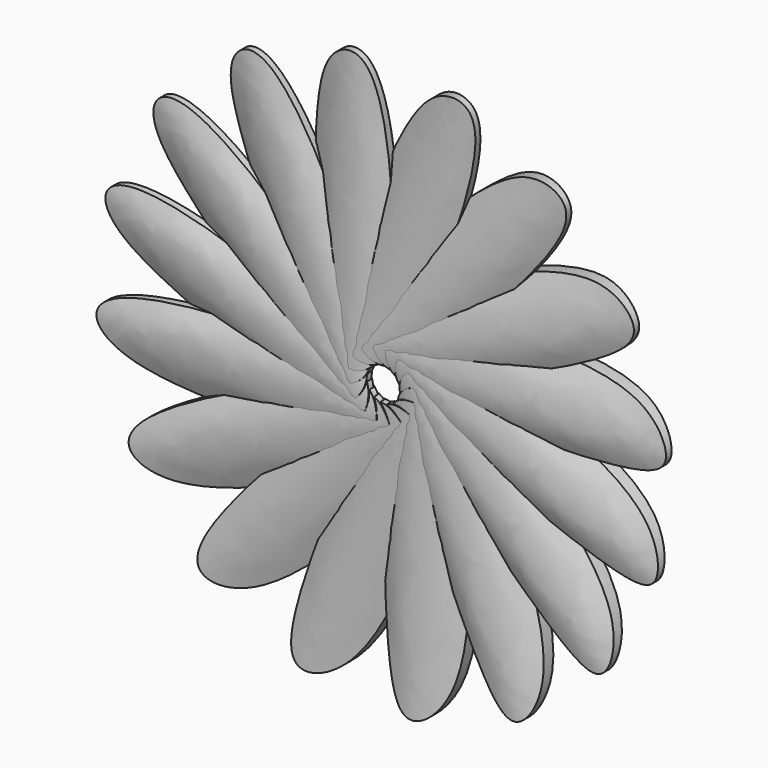
from build123d import *

# Parameters (mm, degrees)
F1_DEPTH = 204
F3_DEPTH = 239
F5_COUNT = 16


with BuildPart() as f1:
    # F0 (on Front) → F1 (new body)
    with BuildSketch(Plane.XZ):
        with BuildLine():
            add(Edge.make_bspline(
                [(-7.4497908354, 168.1414097548), (-10.6516571728, 175.3745122993), (-20.4285228845, 182.9338430563), (-51.5047578624, 156.8177421618), (-47.8448563761, 50.2878389514), (-42.154271715, 4.9962190415), (1.7281079868, -2.3732249511), (4.5337161088, 72.1772189596), (0.5072309671, 150.166282569), (-7.4497908354, 168.1414097548)],
                knots=[0, 0, 0, 0, 0.0807346923, 0.1910522316, 0.4010784068, 0.5334124626, 0.6354068455, 0.7993646083, 1, 1, 1, 1], degree=3))
        make_face()
    extrude(amount=-F1_DEPTH)

    # F2 (on Top) → F3 (intersect)
    with BuildSketch(Plane.XY):
        with BuildLine():
            add(Edge.make_bspline(
                [(39.14796561, 77.6659548283), (39.7631733274, 75.0005164585), (-7.9876774143, -5.9230808558), (-85.7035007244, 65.9992408008), (-85.6405096903, 76.7342301896), (-26.4536337018, 24.2260337862), (10.3763836207, 41.8162409032), (38.6835304134, 79.6781587689), (39.14796561, 77.6659548283)],
                knots=[0, 0, 0, 0, 0.2073158311, 0.4360276951, 0.4754246157, 0.677895944, 0.8434922611, 1, 1, 1, 1], degree=3))
        make_face()
    extrude(amount=F3_DEPTH, mode=Mode.INTERSECT)


with BuildPart() as f5_1:
    # F5: instance of F1
    add(f1.part.rotate(Axis((0, 16.0662084818, 0), (0, 1, 0)), 1 * 360 / F5_COUNT))


with BuildPart() as f5_2:
    # F5: instance of F1
    add(f1.part.rotate(Axis((0, 16.0662084818, 0), (0, 1, 0)), 2 * 360 / F5_COUNT))


with BuildPart() as f5_3:
    # F5: instance of F1
    add(f1.part.rotate(Axis((0, 16.0662084818, 0), (0, 1, 0)), 3 * 360 / F5_COUNT))


with BuildPart() as f5_4:
    # F5: instance of F1
    add(f1.part.rotate(Axis((0, 16.0662084818, 0), (0, 1, 0)), 4 * 360 / F5_COUNT))


with BuildPart() as f5_5:
    # F5: instance of F1
    add(f1.part.rotate(Axis((0, 16.0662084818, 0), (0, 1, 0)), 5 * 360 / F5_COUNT))


with BuildPart() as f5_6:
    # F5: instance of F1
    add(f1.part.rotate(Axis((0, 16.0662084818, 0), (0, 1, 0)), 6 * 360 / F5_COUNT))


with BuildPart() as f5_7:
    # F5: instance of F1
    add(f1.part.rotate(Axis((0, 16.0662084818, 0), (0, 1, 0)), 7 * 360 / F5_COUNT))


with BuildPart() as f5_8:
    # F5: instance of F1
    add(f1.part.rotate(Axis((0, 16.0662084818, 0), (0, 1, 0)), 8 * 360 / F5_COUNT))


with BuildPart() as f5_9:
    # F5: instance of F1
    add(f1.part.rotate(Axis((0, 16.0662084818, 0), (0, 1, 0)), 9 * 360 / F5_COUNT))


with BuildPart() as f5_10:
    # F5: instance of F1
    add(f1.part.rotate(Axis((0, 16.0662084818, 0), (0, 1, 0)), 10 * 360 / F5_COUNT))


with BuildPart() as f5_11:
    # F5: instance of F1
    add(f1.part.rotate(Axis((0, 16.0662084818, 0), (0, 1, 0)), 11 * 360 / F5_COUNT))


with BuildPart() as f5_12:
    # F5: instance of F1
    add(f1.part.rotate(Axis((0, 16.0662084818, 0), (0, 1, 0)), 12 * 360 / F5_COUNT))


with BuildPart() as f5_13:
    # F5: instance of F1
    add(f1.part.rotate(Axis((0, 16.0662084818, 0), (0, 1, 0)), 13 * 360 / F5_COUNT))


with BuildPart() as f5_14:
    # F5: instance of F1
    add(f1.part.rotate(Axis((0, 16.0662084818, 0), (0, 1, 0)), 14 * 360 / F5_COUNT))


with BuildPart() as f5_15:
    # F5: instance of F1
    add(f1.part.rotate(Axis((0, 16.0662084818, 0), (0, 1, 0)), 15 * 360 / F5_COUNT))


solid = Compound([f1.part, f5_1.part, f5_2.part, f5_3.part, f5_4.part, f5_5.part, f5_6.part, f5_7.part, f5_8.part, f5_9.part, f5_10.part, f5_11.part, f5_12.part, f5_13.part, f5_14.part, f5_15.part])
